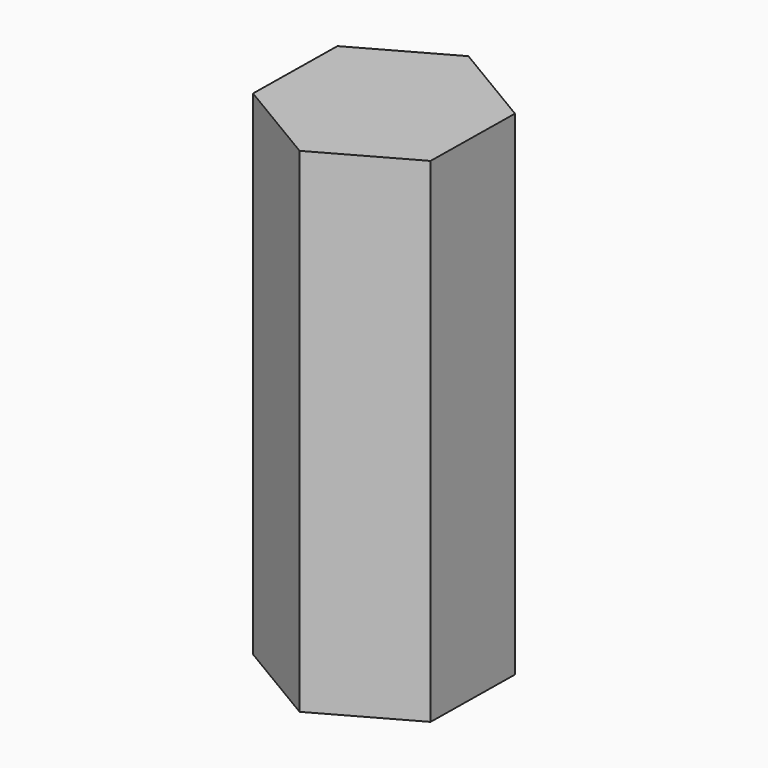
from build123d import *

# Parameters (mm, degrees)
F3_DEPTH = 5.5


# Not quite as in the source:
# - the program builds the solid bodies; features that only make, move or delete a surface that nothing else refers to are left out


with BuildPart() as f3:
    # F2 (on Top) → F3 (new body)
    with BuildSketch(Plane.XY):
        Polygon((1.0081953193, 0.5629169846), (0.0165972508, 1.1545812508), (-0.9915980685, 0.5916642662), (-1.0081953193, -0.5629169846), (-0.0165972508, -1.1545812508), (0.9915980685, -0.5916642662), align=None)
    extrude(amount=-F3_DEPTH)


solid = f3.part
